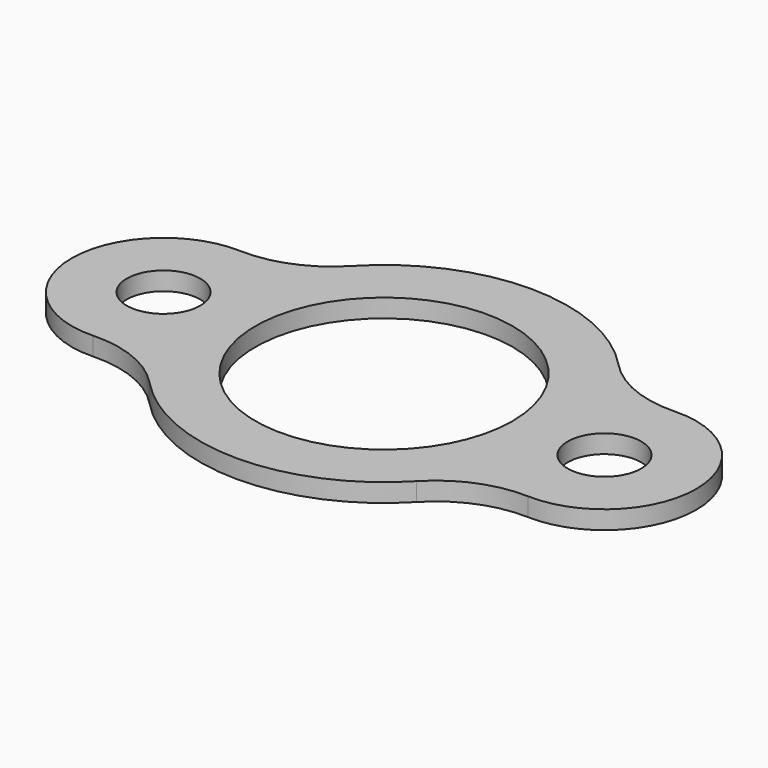
from build123d import *

# Parameters (mm, degrees)
F0_R     = 12.7
F0_R_2   = 44.45
F1_DEPTH = 6.35


# Not quite as in the source:
# - a length typed as a fraction of an inch, garbled in the dataset ("3 / 203.2 mm" for 3/8 in), is restored


with BuildPart() as f1:
    # F0 (on Top) → F1 (new body)
    with BuildSketch(Plane.XY):
        with BuildLine():
            ThreePointArc((-75.1176136364, -31.7315448688), (-59.3475236203, -34.5646316236), (-46.13671875, -43.6308741946))
            ThreePointArc((-46.13671875, -43.6308741946), (0, -63.5), (46.13671875, -43.6308741946))
            ThreePointArc((46.13671875, -43.6308741946), (59.3475236203, -34.5646316236), (75.1176136364, -31.7315448688))
            ThreePointArc((75.1176136364, -31.7315448688), (107.95, 0), (75.1176136364, 31.7315448688))
            ThreePointArc((75.1176136364, 31.7315448688), (59.3475236203, 34.5646316236), (46.13671875, 43.6308741946))
            ThreePointArc((46.13671875, 43.6308741946), (0, 63.5), (-46.13671875, 43.6308741946))
            ThreePointArc((-46.13671875, 43.6308741946), (-59.3475236203, 34.5646316236), (-75.1176136364, 31.7315448688))
            ThreePointArc((-75.1176136364, 31.7315448688), (-107.95, 0), (-75.1176136364, -31.7315448688))
        make_face()
        with Locations((-76.2, 0)):
            Circle(F0_R, mode=Mode.SUBTRACT)
        Circle(F0_R_2, mode=Mode.SUBTRACT)
        with Locations((76.2, 0)):
            Circle(F0_R, mode=Mode.SUBTRACT)
    extrude(amount=F1_DEPTH)


solid = f1.part
